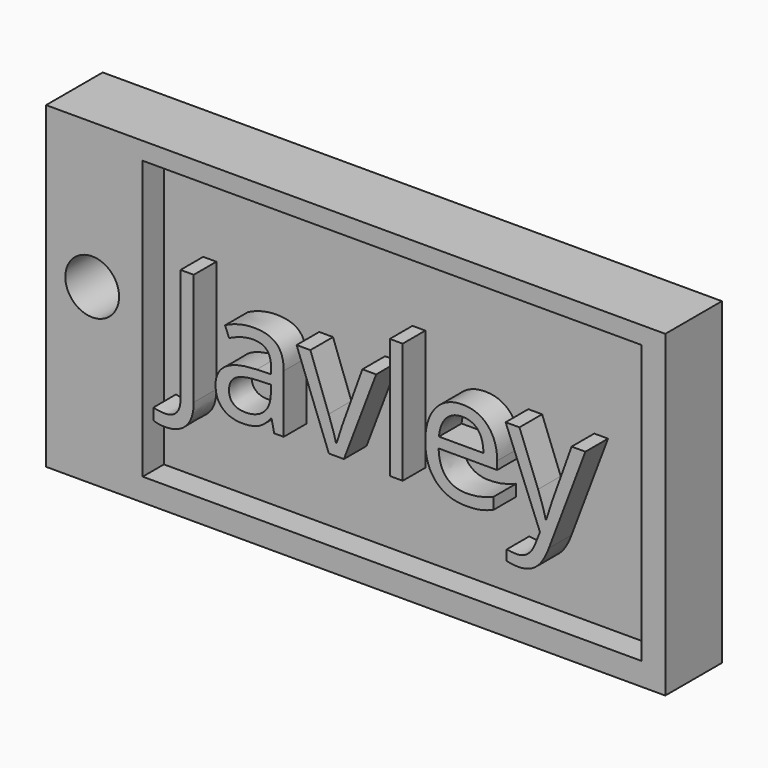
from build123d import *

# Parameters (mm, degrees)
F0_W         = 44.45
F0_H         = 22.86
F0_R         = 1.9289043714
F0_W_2       = 35.8181926422
F0_H_2       = 19.9662228115
F1_DEPTH     = 5.08
F2_DEPTH     = 3.175
F3_TEXT_SIZE = 11.404198002
F4_DEPTH     = 2.032


# Not quite as in the source:
# - Text() gives the source's letters only with a copy of the font that has no kerning and outlines rounded to 1/6400 em; it was checked with that copy


with BuildPart() as f1:
    # F0 (on Front) → F1 (new body)
    with BuildSketch(Plane.XZ):
        with Locations((22.225, 11.43)):
            Rectangle(F0_W, F0_H)
        with Locations((3.3108491916, 12.4531500041)):
            Circle(F0_R, mode=Mode.SUBTRACT)
        with Locations((24.8445069883, 11.6182004567)):
            Rectangle(F0_W_2, F0_H_2, mode=Mode.SUBTRACT)
    extrude(amount=F1_DEPTH)

    # F0 (on Front) → F2 (join)
    with BuildSketch(Plane.XZ):
        with Locations((24.8445069883, 11.6182004567)):
            Rectangle(F0_W_2, F0_H_2)
    extrude(amount=F2_DEPTH)

    # F3 (on face) → F4 (join)
    with BuildSketch(Plane.XZ.offset(3.175)):
        with Locations((8.6965599907, 7.5284014769)):
            Text('Javley', F3_TEXT_SIZE, font='Open Sans', text_align=(TextAlign.LEFT, TextAlign.BOTTOM))
    extrude(amount=F4_DEPTH)


solid = f1.part
